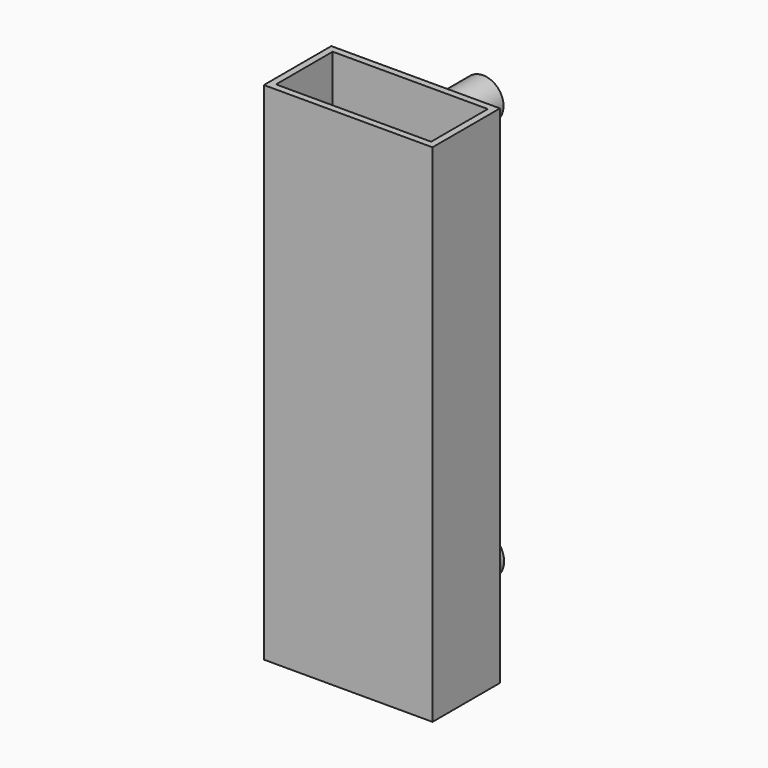
from build123d import *

# Parameters (mm, degrees)
F0_R     = 6.3373
F1_DEPTH = 25.4
F0_R_2   = 6.1645080195
F2_W     = 50.8
F2_H     = 152.4
F3_DEPTH = 25.4
F4_T     = -2.032


# Not quite as in the source:
# - a feature names something its author has since deleted; it is built from what else it names


with BuildPart() as f1:
    # F0 (on Front) → F1 (new body)
    with BuildSketch(Plane.XZ):
        with Locations((0, -60.4431070387)):
            Circle(F0_R)
    extrude(amount=-F1_DEPTH)


with BuildPart() as f1b:
    # F0 (on Front) → F1, piece 2 (new body)
    with BuildSketch(Plane.XZ):
        with Locations((0, 60.2359361947)):
            Circle(F0_R_2)
    extrude(amount=-F1_DEPTH)


with BuildPart() as f3:
    # F2 (on Front) → F3 (new body)
    with BuildSketch(Plane.XZ):
        Rectangle(F2_W, F2_H)
    extrude(amount=F3_DEPTH)

    # F4
    f4_openings = [f3.faces().sort_by_distance(p)[0] for p in [
        (0, -12.7, 76.2),
        (0, -12.7, -76.2),
    ]]
    offset(amount=F4_T, openings=f4_openings)


solid = Compound([f1.part, f1b.part, f3.part])
